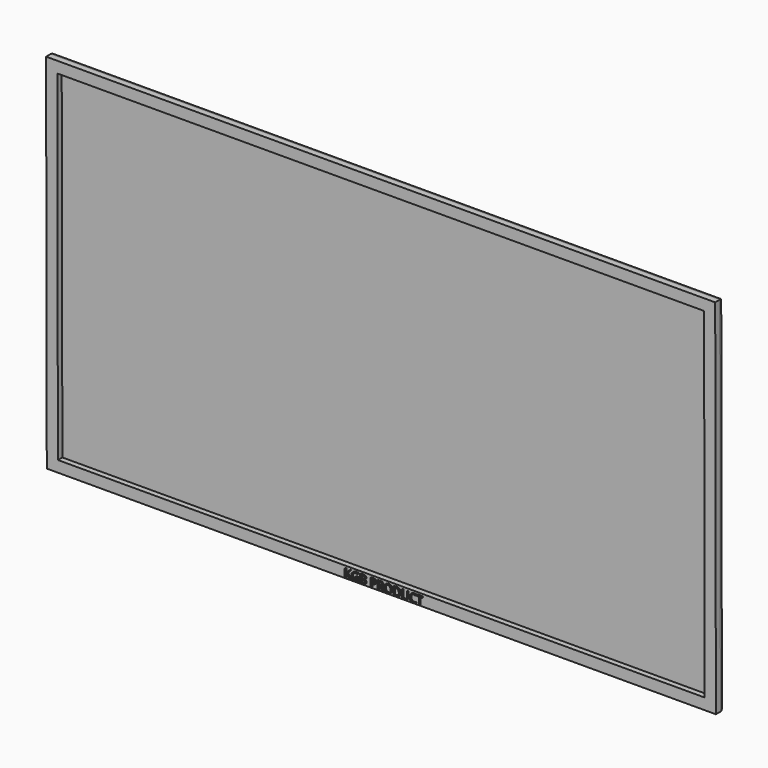
from build123d import *

# Parameters (mm, degrees)
F1_DEPTH     = 10
F2_DEPTH     = 5
F3_TEXT_SIZE = 10.2658238676
F4_DEPTH     = 6
F5_W         = 147.8276401758
F5_H         = 150.907382369
F6_DEPTH     = 10
F7_R         = 15
F8_DEPTH     = 10
F9_R         = 5


# Not quite as in the source:
# - Text() gives the source's letters only with a copy of the font that has no kerning and outlines rounded to 1/6400 em; it was checked with that copy


with BuildPart() as f1:
    # F0 (on Front) → F1 (new body)
    with BuildSketch(Plane.XZ):
        Polygon((300.3136053207, -161.9196975641), (299.6852733497, 163.0796950491), (-300.3136053207, 161.9196975641), (-299.6852733497, -163.0796950491), align=None)
        Polygon((-290.2942907182, 151.9390495444), (289.70462533, 153.0603804465), (290.2942907182, -151.9390495444), (-289.70462533, -153.0603804465), align=None, mode=Mode.SUBTRACT)
    extrude(amount=F1_DEPTH)

    # F0 (on Front) → F2 (join)
    with BuildSketch(Plane.XZ):
        Polygon((290.2942907182, -151.9390495444), (289.70462533, 153.0603804465), (-290.2942907182, 151.9390495444), (-289.70462533, -153.0603804465), align=None)
    extrude(amount=F2_DEPTH)

    # F3 (on face) → F4 (join)
    with BuildSketch(Plane.XZ.offset(5)):
        with Locations((-32.7605456114, -161.5973860025)):
            Text('KGB PRODUCT', F3_TEXT_SIZE, font='Open Sans', text_align=(TextAlign.LEFT, TextAlign.BOTTOM))
    extrude(amount=F4_DEPTH)

    # F5 (on face) → F6 (join)
    with BuildSketch(Plane.XZ):
        with Locations((0.307969749, -0.6159469485)):
            Rectangle(F5_W, F5_H)
    extrude(amount=-F6_DEPTH)

    # F7 (on face) → F8 (cut)
    with BuildSketch(Plane(origin=(0, 10, 0), x_dir=(-1, 0, 0), z_dir=(0, 1, 0))):
        Circle(F7_R)
    extrude(amount=-F8_DEPTH, mode=Mode.SUBTRACT)

    # F9
    f9_edges = [f1.edges().sort_by_distance(p)[0] for p in [
        (0.30797, 0, 74.837744),
        (74.22179, 0, -0.615947),
        (0.30797, 0, -76.069638),
        (299.999439, 0, 0.579999),
        (0.314166, 0, -162.499696),
        (-0.314166, 0, 162.499696),
        (-299.999439, 0, -0.579999),
        (-73.60585, 0, -0.615947),
    ]]
    fillet(f9_edges, radius=F9_R)


solid = f1.part
